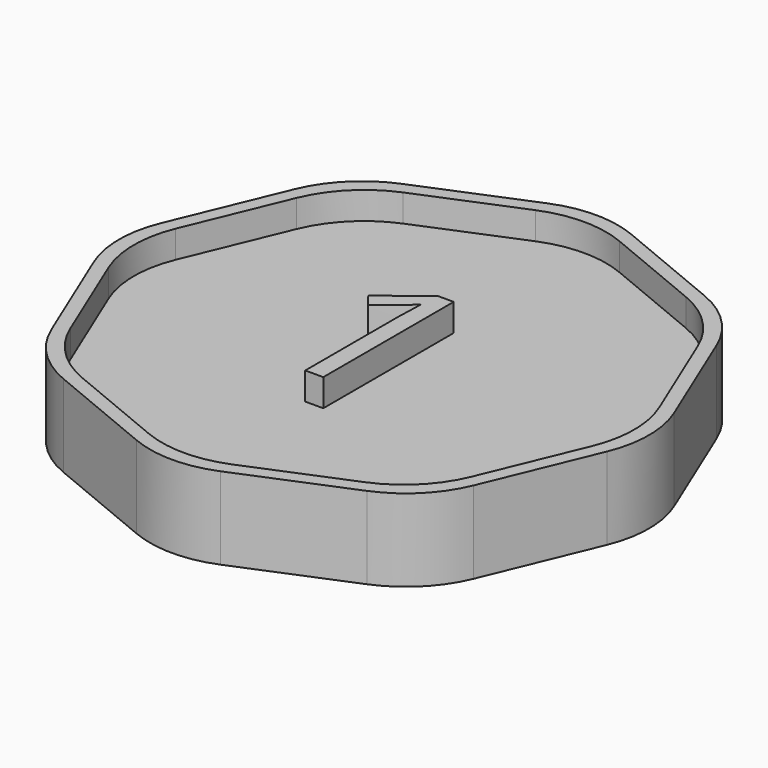
from build123d import *

# Parameters (mm, degrees)
F3_DEPTH     = 3
F5_DEPTH     = 1
F7_DEPTH     = 1
F8_TEXT_SIZE = 8.3333333333
F9_DEPTH     = 1
F11_DEPTH    = 1


# Not quite as in the source:
# - Text() gives the source's letters only with a copy of the font that has no kerning and outlines rounded to 1/6400 em; it was checked with that copy


with BuildPart() as f3:
    # F2 (on Top) → F3 (new body)
    with BuildSketch(Plane.XY):
        with BuildLine():
            Line((7.705118483, -5.5403340824), (9.3659493289, -1.5307337295))
            ThreePointArc((9.3659493289, -1.5307337295), (9.6704311988, 0), (9.3659493289, 1.5307337295))
            Line((9.3659493289, 1.5307337295), (7.705118483, 5.5403340824))
            ThreePointArc((7.705118483, 5.5403340824), (6.8380274777, 6.8380274777), (5.5403340824, 7.705118483))
            Line((5.5403340824, 7.705118483), (1.5307337295, 9.3659493289))
            ThreePointArc((1.5307337295, 9.3659493289), (0, 9.6704311988), (-1.5307337295, 9.3659493289))
            Line((-1.5307337295, 9.3659493289), (-5.5403340824, 7.705118483))
            ThreePointArc((-5.5403340824, 7.705118483), (-6.8380274777, 6.8380274777), (-7.705118483, 5.5403340824))
            Line((-7.705118483, 5.5403340824), (-9.3659493289, 1.5307337295))
            ThreePointArc((-9.3659493289, 1.5307337295), (-9.6704311988, 0), (-9.3659493289, -1.5307337295))
            Line((-9.3659493289, -1.5307337295), (-7.705118483, -5.5403340824))
            ThreePointArc((-7.705118483, -5.5403340824), (-6.8380274777, -6.8380274777), (-5.5403340824, -7.705118483))
            Line((-5.5403340824, -7.705118483), (-1.5307337295, -9.3659493289))
            ThreePointArc((-1.5307337295, -9.3659493289), (0, -9.6704311988), (1.5307337295, -9.3659493289))
            Line((1.5307337295, -9.3659493289), (5.5403340824, -7.705118483))
            ThreePointArc((5.5403340824, -7.705118483), (6.8380274777, -6.8380274777), (7.705118483, -5.5403340824))
        make_face()
    extrude(amount=-F3_DEPTH)

    # F4 (on face) → F5 (cut)
    with BuildSketch(Plane.XY):
        with BuildLine():
            Line((-8.8247532287, -1.5307337295), (-7.3224350506, -5.15765065))
            ThreePointArc((-7.3224350506, -5.15765065), (-6.4553440453, -6.4553440453), (-5.15765065, -7.3224350506))
            Line((-5.15765065, -7.3224350506), (-1.5307337295, -8.8247532287))
            ThreePointArc((-1.5307337295, -8.8247532287), (0, -9.1292350987), (1.5307337295, -8.8247532287))
            Line((1.5307337295, -8.8247532287), (5.15765065, -7.3224350506))
            ThreePointArc((5.15765065, -7.3224350506), (6.4553440453, -6.4553440453), (7.3224350506, -5.15765065))
            Line((7.3224350506, -5.15765065), (8.8247532287, -1.5307337295))
            ThreePointArc((8.8247532287, -1.5307337295), (9.1292350987, 0), (8.8247532287, 1.5307337295))
            Line((8.8247532287, 1.5307337295), (7.3224350506, 5.15765065))
            ThreePointArc((7.3224350506, 5.15765065), (6.4553440453, 6.4553440453), (5.15765065, 7.3224350506))
            Line((5.15765065, 7.3224350506), (1.5307337295, 8.8247532287))
            ThreePointArc((1.5307337295, 8.8247532287), (0, 9.1292350987), (-1.5307337295, 8.8247532287))
            Line((-1.5307337295, 8.8247532287), (-5.15765065, 7.3224350506))
            ThreePointArc((-5.15765065, 7.3224350506), (-6.4553440453, 6.4553440453), (-7.3224350506, 5.15765065))
            Line((-7.3224350506, 5.15765065), (-8.8247532287, 1.5307337295))
            ThreePointArc((-8.8247532287, 1.5307337295), (-9.1292350987, 0), (-8.8247532287, -1.5307337295))
        make_face()
    extrude(amount=-F5_DEPTH, mode=Mode.SUBTRACT)

    # F6 (on face) → F7 (cut)
    with BuildSketch(Plane(origin=(0, 0, -3), x_dir=(1, 0, 0), z_dir=(0, 0, -1))):
        with BuildLine():
            ThreePointArc((-8.8247532287, 1.5307337295), (-9.1292350987, 0), (-8.8247532287, -1.5307337295))
            Line((-8.8247532287, -1.5307337295), (-7.3224350506, -5.15765065))
            ThreePointArc((-7.3224350506, -5.15765065), (-6.4553440453, -6.4553440453), (-5.15765065, -7.3224350506))
            Line((-5.15765065, -7.3224350506), (-1.5307337295, -8.8247532287))
            ThreePointArc((-1.5307337295, -8.8247532287), (0, -9.1292350987), (1.5307337295, -8.8247532287))
            Line((1.5307337295, -8.8247532287), (5.15765065, -7.3224350506))
            ThreePointArc((5.15765065, -7.3224350506), (6.4553440453, -6.4553440453), (7.3224350506, -5.15765065))
            Line((7.3224350506, -5.15765065), (8.8247532287, -1.5307337295))
            ThreePointArc((8.8247532287, -1.5307337295), (9.1292350987, 0), (8.8247532287, 1.5307337295))
            Line((8.8247532287, 1.5307337295), (7.3224350506, 5.15765065))
            ThreePointArc((7.3224350506, 5.15765065), (6.4553440453, 6.4553440453), (5.15765065, 7.3224350506))
            Line((5.15765065, 7.3224350506), (1.5307337295, 8.8247532287))
            ThreePointArc((1.5307337295, 8.8247532287), (0, 9.1292350987), (-1.5307337295, 8.8247532287))
            Line((-1.5307337295, 8.8247532287), (-5.15765065, 7.3224350506))
            ThreePointArc((-5.15765065, 7.3224350506), (-6.4553440453, 6.4553440453), (-7.3224350506, 5.15765065))
            Line((-7.3224350506, 5.15765065), (-8.8247532287, 1.5307337295))
        make_face()
    extrude(amount=-F7_DEPTH, mode=Mode.SUBTRACT)

    # F8 (on face) → F9 (join)
    with BuildSketch(Plane.XY.offset(-1)):
        with Locations((-2.724609375, -3)):
            Text('1', F8_TEXT_SIZE, font='Open Sans', text_align=(TextAlign.LEFT, TextAlign.BOTTOM))
    extrude(amount=F9_DEPTH)

    # F10 (on face) → F11 (join)
    with BuildSketch(Plane(origin=(0, 0, -2), x_dir=(1, 0, 0), z_dir=(0, 0, -1))):
        with BuildLine():
            Line((0.9201765066, 4.3568853246), (0, 2.1890853246))
            Line((0, 2.1890853246), (-0.9201765066, 4.3568853246))
            Line((-0.9201765066, 4.3568853246), (-3.4873365066, 4.3568853246))
            Line((-3.4873365066, 4.3568853246), (-1.9853663274, 0.8184653246))
            add(Edge.make_bspline(
                [(-1.9853663274, 0.8184653246), (-2.86118, 0.6846253246), (-4.3868581819, 0.5563170367), (-6.0514905321, -0.4962494273), (-2.7779407391, -1.7882286366), (-1.8097922734, -1.5925497793), (-1.6920312198, -3.6039368733), (-0.6283421363, -4.5636769026), (-0.17888, -4.5824246754), (0, -4.5824246754)],
                knots=[0, 0, 0, 0, 0.1906946011, 0.3116321419, 0.5087037577, 0.6185878054, 0.772744227, 0.9107655949, 1, 1, 1, 1], degree=3))
            add(Edge.make_bspline(
                [(1.9853663274, 0.8184653246), (2.86118, 0.6846253246), (4.3868581819, 0.5563170367), (6.0514905321, -0.4962494273), (2.7779407391, -1.7882286366), (1.8097922734, -1.5925497793), (1.6920312198, -3.6039368733), (0.6283421363, -4.5636769026), (0.17888, -4.5824246754), (0, -4.5824246754)],
                knots=[0, 0, 0, 0, 0.1906946011, 0.3116321419, 0.5087037577, 0.6185878054, 0.772744227, 0.9107655949, 1, 1, 1, 1], degree=3))
            Line((1.9853663274, 0.8184653246), (3.4873365066, 4.3568853246))
            Line((3.4873365066, 4.3568853246), (0.9201765066, 4.3568853246))
        make_face()
    extrude(amount=F11_DEPTH)


solid = f3.part
